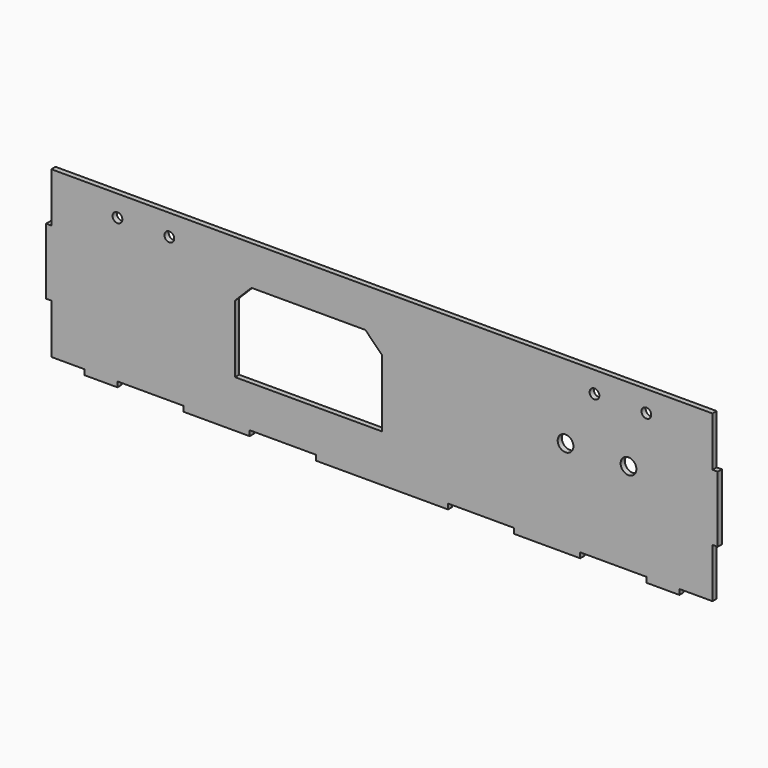
from build123d import *

# Parameters (mm, degrees)
F0_R     = 1.4732
F0_R_2   = 2.38125
F0_W     = 1.5875
F0_H     = 20
F0_W_2   = 10
F0_H_2   = 1.5875
F0_W_3   = 20
F1_DEPTH = 1.5875
F2_SIZE  = 5


# Not quite as in the source:
# - a length typed as a fraction of an inch, garbled in the dataset ("3 / 203.2 mm" for 3/8 in), is restored


with BuildPart() as f1:
    # F0 (on Front) → F1 (new body)
    with BuildSketch(Plane.XZ):
        Polygon((100, 10), (100, 25), (-100, 25), (-100, 10), (-100, -10), (-100, -25), (-90, -25), (-80, -25), (-60, -25), (-44.45, -25), (-44.45, -12.3), (-44.45, 13.1), (0, 13.1), (0, -12.3), (0, -25), (20, -25), (40, -25), (60, -25), (80, -25), (90, -25), (100, -25), (100, -10), align=None)
        with Locations((-80, 18.6)):
            Circle(F0_R, mode=Mode.SUBTRACT)
        with Locations((-64.3028, 18.6)):
            Circle(F0_R, mode=Mode.SUBTRACT)
        with Locations((55.55, 2.5678405073)):
            Circle(F0_R_2, mode=Mode.SUBTRACT)
        with Locations((74.6, 2.6706890203)):
            Circle(F0_R_2, mode=Mode.SUBTRACT)
        with Locations((64.3028, 18.6)):
            Circle(F0_R, mode=Mode.SUBTRACT)
        with Locations((80, 18.6)):
            Circle(F0_R, mode=Mode.SUBTRACT)
        with Locations((100.79375, 0)):
            Rectangle(F0_W, F0_H)
        with Locations((-100.79375, 0)):
            Rectangle(F0_W, F0_H)
        with Locations((85, -25.79375)):
            Rectangle(F0_W_2, F0_H_2)
        with Locations((-85, -25.79375)):
            Rectangle(F0_W_2, F0_H_2)
        with Locations((50, -25.79375)):
            Rectangle(F0_W_3, F0_H_2)
        Polygon((-44.45, -25), (-60, -25), (-60, -26.5875), (-40, -26.5875), (-40, -25), align=None)
        Polygon((-44.45, -12.3), (-44.45, -25), (-40, -25), (-20, -25), (0, -25), (0, -12.3), align=None)
        Polygon((20, -26.5875), (20, -25), (0, -25), (-20, -25), (-20, -26.5875), align=None)
    extrude(amount=F1_DEPTH)

    # F2
    f2_edges = [f1.edges().sort_by_distance(p)[0] for p in [
        (-44.45, -0.79375, 13.1),
        (0, -0.79375, 13.1),
    ]]
    chamfer(f2_edges, length=F2_SIZE)


solid = f1.part
